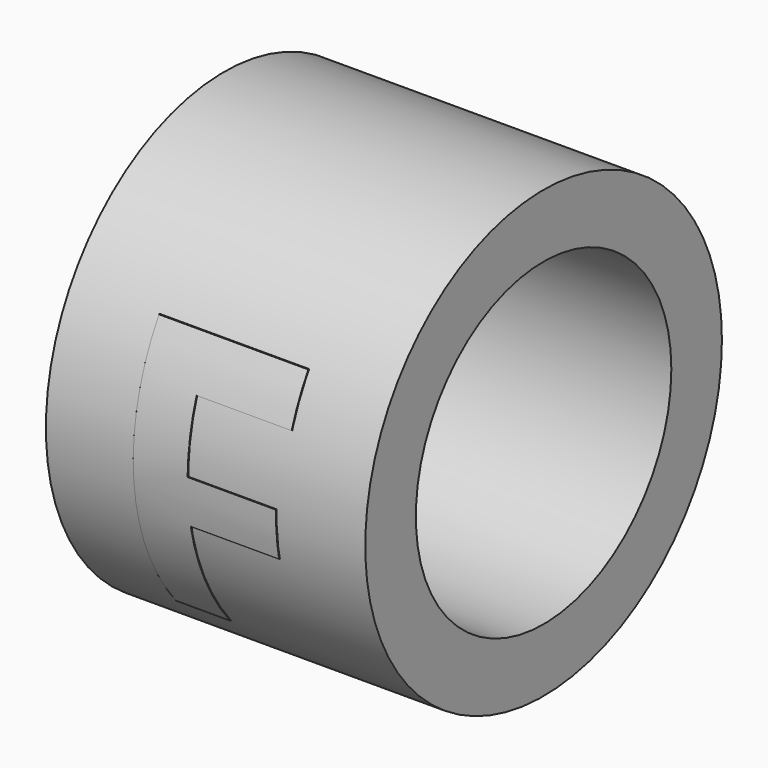
from build123d import *

# Parameters (mm, degrees)
F0_R         = 1.75
F0_R_2       = 1.745
F0_R_3       = 1.25
F1_DEPTH     = 2.5
F2_TEXT_SIZE = 2.8570699214
F3_REACH     = 4.1020094213
F4_DEPTH     = 2.5


# Not quite as in the source:
# - Text() gives the source's letters only with a copy of the font that has no kerning and outlines rounded to 1/6400 em; it was checked with that copy


with BuildPart() as f1:
    # F0 (on Right) → F1 (new body)
    with BuildSketch(Plane.YZ):
        Circle(F0_R)
        Circle(F0_R_2, mode=Mode.SUBTRACT)
        Circle(F0_R_2)
        Circle(F0_R_3, mode=Mode.SUBTRACT)
    extrude(amount=F1_DEPTH)

    f3_end = f1.faces().sort_by_distance((1.25, -1.75, 0))[0]
    # F2 (on Front) → F3 (intersect, up to a face of the model that its end follows)
    with BuildSketch(Plane.XZ):
        with Locations((0.4309935612, -1.1343103251)):
            Text('F', F2_TEXT_SIZE, font='Open Sans', font_style=FontStyle.BOLD, text_align=(TextAlign.LEFT, TextAlign.BOTTOM))
    f3_long = extrude(amount=F3_REACH, mode=Mode.PRIVATE)
    add(split(f3_long, bisect_by=f3_end, keep=Keep.BOTTOM, mode=Mode.PRIVATE), mode=Mode.INTERSECT)


with BuildPart() as f4:
    # F0 (on Right) → F4 (new body)
    with BuildSketch(Plane.YZ):
        Circle(F0_R_2)
        Circle(F0_R_3, mode=Mode.SUBTRACT)
    extrude(amount=F4_DEPTH)


solid = Compound([f1.part, f4.part])
